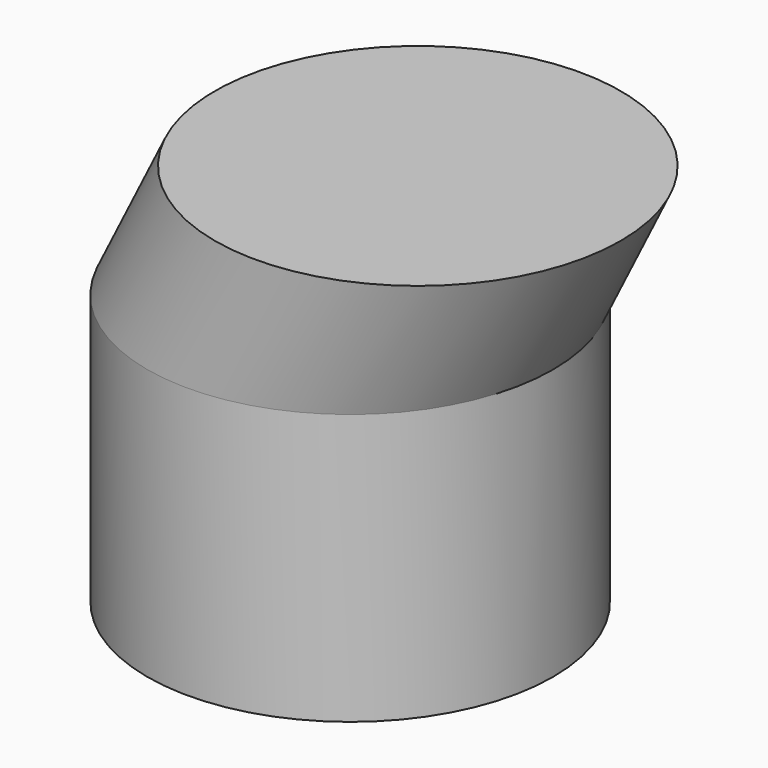
from build123d import *

# Parameters (mm, degrees)
F0_R     = 19.05
F1_DEPTH = 25.4
F4_R     = 19.05
F3_R     = 19.05


with BuildPart() as f1:
    # F0 (on Top) → F1 (new body)
    with BuildSketch(Plane.XY):
        Circle(F0_R)
    extrude(amount=F1_DEPTH)


with BuildPart() as f7:
    # F4 (on face) → F7 section 0
    with BuildSketch(Plane.XY.offset(25.4)):
        Circle(F4_R)
    # F3 (on offset) → F7 section 1
    with BuildSketch(Plane.XY.offset(38.1)):
        with Locations((6.35, 0)):
            Circle(F3_R)
    loft()


solid = Compound([f1.part, f7.part])
